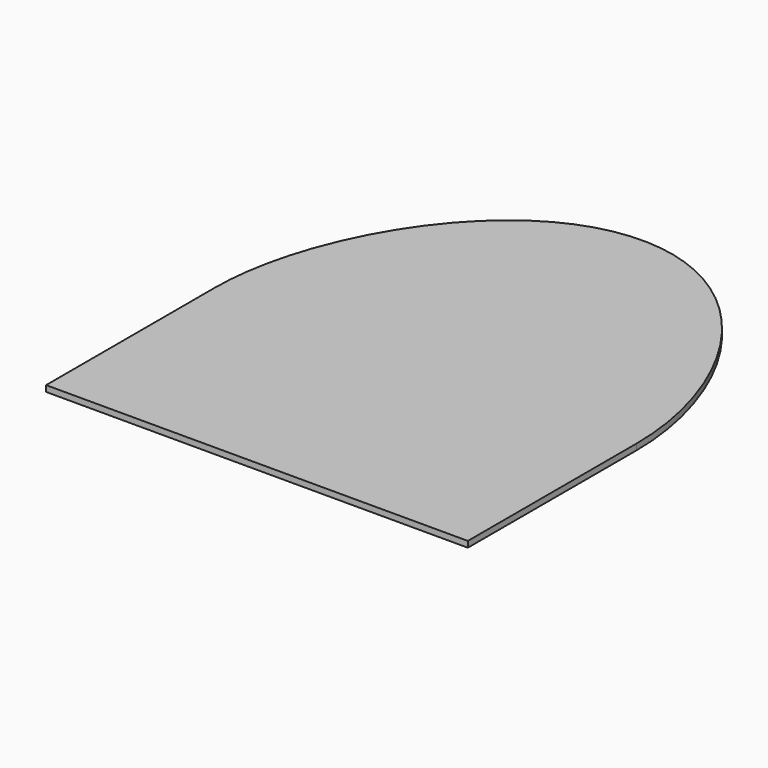
from build123d import *

# Parameters (mm, degrees)
F1_DEPTH = 1


# Not quite as in the source:
# - ends of sketch curves that miss each other by under 0.0002 mm in the source are joined


with BuildPart() as f1:
    # F0 (on Top) → F1 (new body)
    with BuildSketch(Plane.XY):
        with BuildLine():
            Line((-35, 2.1762e-06), (-35, -35))
            Line((-35, -35), (-27, -35))
            Line((-27, -35), (-27, -22.2710574513))
            ThreePointArc((-27, -22.2710574513), (-32.9393385518, -11.8321585422), (-35, 2.1762e-06))
        make_face()
        with BuildLine():
            Line((-27, -22.2710574513), (-27, -35))
            Line((-27, -35), (1.91e-08, -35))
            ThreePointArc((1.91e-08, -35), (-14.9250291237, -31.6582296671), (-27, -22.2710574513))
        make_face()
        with BuildLine():
            add(Edge.make_bspline(
                [(0, 45), (-20.1986748725, 45), (-35, 20.0504870868), (-35, 2.1762e-06)],
                knots=[0, 0, 0, 0, 57.0087695372, 57.0087695372, 57.0087695372, 57.0087695372], degree=3))
            ThreePointArc((-35, 2.1762e-06), (-28.4666369261, 20.3629708568), (-11.3056830814, 33.1237306181))
            ThreePointArc((-11.3056830814, 33.1237306181), (20.3629699719, 28.4666375592), (35, 0))
            add(Edge.make_bspline(
                [(0, 45), (20.1986748725, 45), (35, 20.0504870868), (35, 0)],
                knots=[0, 0, 0, 0, 57.0087695372, 57.0087695372, 57.0087695372, 57.0087695372], degree=3))
        make_face()
        with BuildLine():
            ThreePointArc((-11.3056830814, 33.1237306181), (-28.4666369261, 20.3629708568), (-35, 2.1762e-06))
            ThreePointArc((-35, 2.1762e-06), (-32.9393385518, -11.8321585422), (-27, -22.2710574513))
            Line((-27, -22.2710574513), (-27, 2.1762e-06))
            add(Edge.make_bspline(
                [(-11.3056830814, 33.1237306181), (-12.4097508436, 32.3488132243), (-15.1414824386, 30.0752135158), (-18.8876274503, 25.5283101279), (-22.422035633, 19.604279738), (-25.0662594291, 13.1120426553), (-26.6478130576, 7.1844788974), (-27.0173066601, 2.7756083867), (-27.018694794, 0.6711028041), (-27, 2.1762e-06)],
                knots=[12.1476935207, 12.1476935207, 12.1476935207, 12.1476935207, 16.189226149, 22.7543847852, 29.7183326598, 36.8091409701, 43.7289829573, 48.0262708445, 50.0404462243, 50.0404462243, 50.0404462243, 50.0404462243], degree=3))
        make_face()
        with BuildLine():
            ThreePointArc((35, 0), (24.7487373483, -24.7487373348), (1.91e-08, -35))
            Line((1.91e-08, -35), (35, -35))
            Line((35, -35), (35, 0))
        make_face()
        with BuildLine():
            ThreePointArc((-27, -22.2710574513), (-14.9250291237, -31.6582296671), (1.91e-08, -35))
            ThreePointArc((1.91e-08, -35), (24.7487373483, -24.7487373348), (35, 0))
            ThreePointArc((35, 0), (20.3629699719, 28.4666375592), (-11.3056830814, 33.1237306181))
            add(Edge.make_bspline(
                [(-11.3056830814, 33.1237306181), (-12.4097508436, 32.3488132243), (-15.1414824386, 30.0752135158), (-18.8876274503, 25.5283101279), (-22.422035633, 19.604279738), (-25.0662594291, 13.1120426553), (-26.6478130576, 7.1844788974), (-27.0173066601, 2.7756083867), (-27.018694794, 0.6711028041), (-27, 2.1762e-06)],
                knots=[12.1476935207, 12.1476935207, 12.1476935207, 12.1476935207, 16.189226149, 22.7543847852, 29.7183326598, 36.8091409701, 43.7289829573, 48.0262708445, 50.0404462243, 50.0404462243, 50.0404462243, 50.0404462243], degree=3))
            Line((-27, 2.1762e-06), (-27, -22.2710574513))
        make_face()
    extrude(amount=F1_DEPTH)


solid = f1.part
